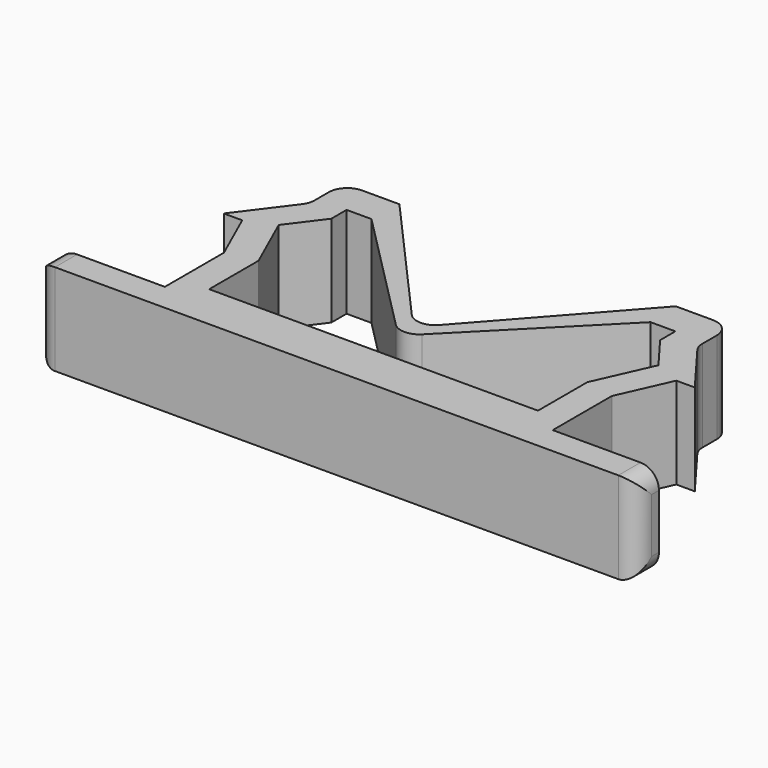
from build123d import *

# Parameters (mm, degrees)
F1_DEPTH = 4.95
F2_R     = 1


with BuildPart() as f1:
    # F0 (on Top) → F1 (new body)
    with BuildSketch(Plane.XY):
        Polygon((-16.25, 0), (0, 0), (16.25, 0), (16.25, 1.5), (10.5, 1.5), (10.5, 5.5), (11.75, 8.3), (12.75, 8.3), (10.5, 11.3), (10.5, 13.6000004441), (7.4805053882, 13.6000004441), (0, 5.1791056932), (-7.4805053882, 13.6000004441), (-10.5, 13.6000004441), (-10.5, 11.3), (-12.75, 8.3), (-11.75, 8.3), (-10.5, 5.5), (-10.5, 1.5), (-16.25, 1.5), align=None)
        Polygon((-10.2784717774, 8.9287042967), (-8.9, 10.7666666667), (-8.9, 11.8000004441), (-7.5543964098, 11.8000004441), (0, 4.1791056932), (7.5543964098, 11.8000004441), (8.9, 11.8000004441), (8.9, 10.7666666667), (10.2784717774, 8.9287042967), (8.9, 5.8409275153), (8.9, 2.5), (0, 2.5), (-8.9, 2.5), (-8.9, 5.8409275153), align=None, mode=Mode.SUBTRACT)
    extrude(amount=F1_DEPTH)

    # F2
    f2_edges = [f1.edges().sort_by_distance(p)[0] for p in [
        (-16.25, 0.75, 4.95),
        (-16.25, 0.75, 0),
        (16.25, 0.75, 4.95),
        (16.25, 0.75, 0),
        (-16.25, 0, 2.475),
        (16.25, 0, 2.475),
        (0, 5.179106, 2.475),
        (0, 4.179106, 2.475),
        (-10.5, 11.3, 2.475),
        (-10.5, 13.6, 2.475),
        (10.5, 13.6, 2.475),
        (10.5, 11.3, 2.475),
    ]]
    fillet(f2_edges, radius=F2_R)


solid = f1.part
